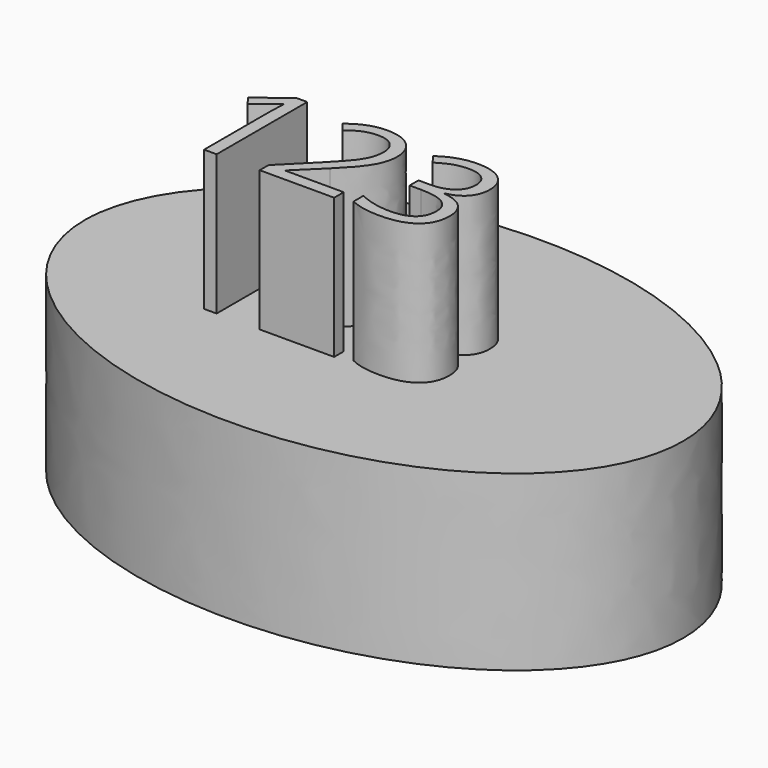
from build123d import *

# Parameters (mm, degrees)
F1_DEPTH     = 35.814
F2_TEXT_SIZE = 32.7731909541
F3_DEPTH     = 28.956


# Not quite as in the source:
# - Text() gives the source's letters only with a copy of the font that has no kerning and outlines rounded to 1/6400 em; it was checked with that copy


with BuildPart() as f1:
    # F0 (on Top) → F1 (new body)
    with BuildSketch(Plane.XY):
        with BuildLine():
            add(Edge.make_bspline(
                [(-61.8166327477, 0), (-61.8166327477, -70.1575525678), (30.9083163738, -35.0787762839), (123.6332654953, 0), (30.9083163738, 35.0787762839), (-61.8166327477, 70.1575525678), (-61.8166327477, 0)],
                knots=[0, 0, 0, 2.0943951024, 2.0943951024, 4.1887902048, 4.1887902048, 6.2831853072, 6.2831853072, 6.2831853072], degree=2, weights=[1, 0.5, 1, 0.5, 1, 0.5, 1]))
        make_face()
    extrude(amount=F1_DEPTH)


with BuildPart() as f3:
    # F2 (on face) → F3 (new body)
    with BuildSketch(Plane.XY.offset(35.814)):
        with Locations((-36.2402722239, -12.212314643)):
            Text('123', F2_TEXT_SIZE, font='Open Sans', text_align=(TextAlign.LEFT, TextAlign.BOTTOM))
    extrude(amount=F3_DEPTH)


solid = Compound([f1.part, f3.part])
